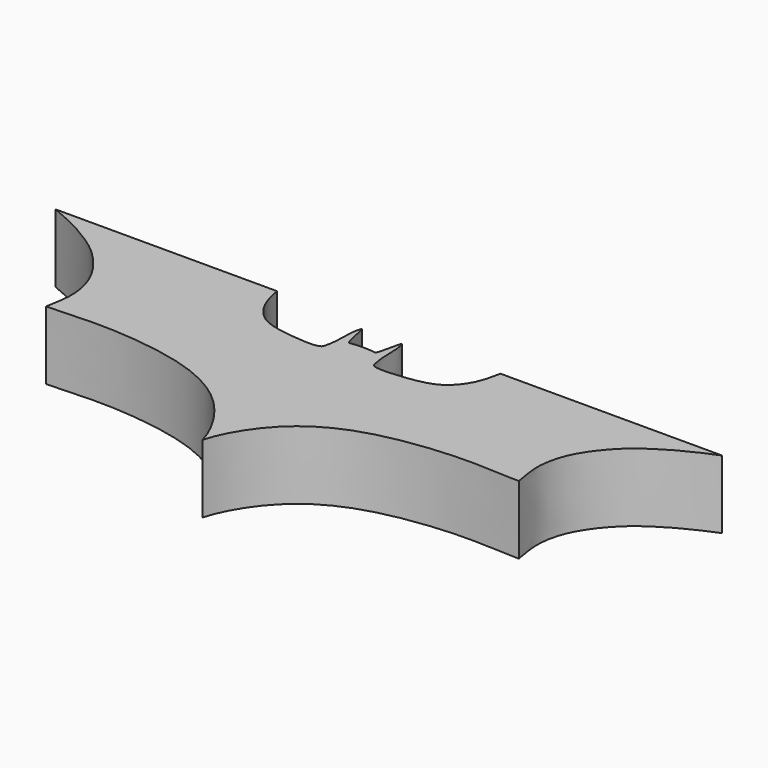
from build123d import *

# Parameters (mm, degrees)
F1_DEPTH = 10


with BuildPart() as f1:
    # F0 (on Top) → F1 (new body)
    with BuildSketch(Plane.XY):
        with BuildLine():
            add(Edge.make_bspline(
                [(-34.5659777522, -2.3010377772), (-34.441690892, -1.2090269011), (-33.7426143908, 1.3021229087), (-34.6099625003, 6.2887083902), (-37.732299485, 10.4337765544), (-40.4965689238, 12.9182984992), (-45.1676660532, 15.6816198367), (-47.6433440327, 16.6521064837), (-48.734344542, 17.1325933188)],
                knots=[0, 0, 0, 0, 0.1504717907, 0.3274056637, 0.505806187, 0.6605615473, 0.844008032, 1, 1, 1, 1], degree=3))
            add(Edge.make_bspline(
                [(-34.5659777522, -2.3010377772), (-29.7742336988, -2.0793164149), (-24.8478324902, -1.8245382393), (-12.9343956026, -3.3284422394), (-4.2994288291, -8.106275212), (-0.6981744502, -14.3344540986), (0, -16.8964266777)],
                knots=[0, 0, 0, 0, 0.2532524451, 0.514284306, 0.7614910609, 1, 1, 1, 1], degree=3))
            add(Edge.make_bspline(
                [(34.5659777522, -2.3010377772), (29.7742336988, -2.0793164149), (24.8478324902, -1.8245382393), (12.9343956026, -3.3284422394), (4.2994288291, -8.106275212), (0.6981744502, -14.3344540986), (0, -16.8964266777)],
                knots=[0, 0, 0, 0, 0.2532524451, 0.514284306, 0.7614910609, 1, 1, 1, 1], degree=3))
            add(Edge.make_bspline(
                [(34.5659777522, -2.3010377772), (34.441690892, -1.2090269011), (33.7426143908, 1.3021229087), (34.6099625003, 6.2887083902), (37.732299485, 10.4337765544), (40.4965689238, 12.9182984992), (45.1676660532, 15.6816198367), (47.6433440327, 16.6521064837), (48.734344542, 17.1325933188)],
                knots=[0, 0, 0, 0, 0.1504717907, 0.3274056637, 0.505806187, 0.6605615473, 0.844008032, 1, 1, 1, 1], degree=3))
            Line((48.734344542, 17.1325933188), (16.3374114782, 17.1325933188))
            add(Edge.make_bspline(
                [(16.3374114782, 17.1325933188), (16.2707590578, 16.8013167715), (16.1028193617, 16.0159047713), (15.5293351039, 13.5894216644), (13.5075885145, 10.9357028955), (11.0943832685, 9.979418199), (8.3278162532, 9.4999515323), (4.2337515187, 9.1916813282), (3.7513867907, 9.7417653506), (3.721309654, 9.7951889602)],
                knots=[0, 0, 0, 0, 0.1002529863, 0.2510752424, 0.4252888894, 0.575274046, 0.7448218724, 0.9396020225, 0.9846016995, 0.9846016995, 0.9846016995, 0.9846016995], degree=3))
            Line((3.721309654, 9.7951889602), (3.6973344953, 9.8154297664))
            add(Edge.make_bspline(
                [(2.932772506, 15.9026999027), (3.018619719, 15.6514358008), (3.2073644933, 15.0990033508), (3.3168408961, 13.9617858734), (3.3565401619, 12.068204215), (3.4100837285, 11.0186767215), (3.599767527, 10.2241220004), (3.6973344953, 9.8154297664)],
                knots=[0, 0, 0, 0, 0.16399089, 0.3605524565, 0.6106599974, 0.7997365931, 1, 1, 1, 1], degree=3))
            add(Edge.make_bspline(
                [(2.932772506, 15.9026999027), (2.8831992541, 15.7815790305), (2.7595296769, 15.4794207803), (2.6079557623, 14.5179694226), (2.311756701, 13.4620564486), (2.1469901884, 12.6659080553), (2.0074066607, 12.3726247092), (1.9479012117, 12.2475959361)],
                knots=[0, 0, 0, 0, 0.1539432383, 0.3840396681, 0.6350969803, 0.8444392514, 1, 1, 1, 1], degree=3))
            add(Edge.make_bspline(
                [(1.9479012117, 12.2475959361), (1.7516233528, 12.2796352379), (1.3532942381, 12.3446562585), (0.7217223004, 12.418893829), (0.2458943028, 12.4186232246), (0, 12.418483384)],
                knots=[0, 0, 0, 0, 0.3194597762, 0.6483162725, 1, 1, 1, 1], degree=3))
            add(Edge.make_bspline(
                [(-1.9479012117, 12.2475959361), (-1.7516233528, 12.2796352379), (-1.3532942381, 12.3446562585), (-0.7217223004, 12.418893829), (-0.2458943028, 12.4186232246), (0, 12.418483384)],
                knots=[0, 0, 0, 0, 0.3194597762, 0.6483162725, 1, 1, 1, 1], degree=3))
            add(Edge.make_bspline(
                [(-2.932772506, 15.9026999027), (-2.8831992541, 15.7815790305), (-2.7595296769, 15.4794207803), (-2.6079557623, 14.5179694226), (-2.311756701, 13.4620564486), (-2.1469901884, 12.6659080553), (-2.0074066607, 12.3726247092), (-1.9479012117, 12.2475959361)],
                knots=[0, 0, 0, 0, 0.1539432383, 0.3840396681, 0.6350969803, 0.8444392514, 1, 1, 1, 1], degree=3))
            add(Edge.make_bspline(
                [(-2.932772506, 15.9026999027), (-3.018619719, 15.6514358008), (-3.2073644933, 15.0990033508), (-3.3168408961, 13.9617858734), (-3.3565401619, 12.068204215), (-3.4100837285, 11.0186767215), (-3.599767527, 10.2241220004), (-3.6973344953, 9.8154297664)],
                knots=[0, 0, 0, 0, 0.16399089, 0.3605524565, 0.6106599974, 0.7997365931, 1, 1, 1, 1], degree=3))
            Line((-3.6973344953, 9.8154297664), (-3.721309654, 9.7951889602))
            add(Edge.make_bspline(
                [(-16.3374114782, 17.1325933188), (-16.2707590578, 16.8013167715), (-16.1028193617, 16.0159047713), (-15.5293351039, 13.5894216644), (-13.5075885145, 10.9357028955), (-11.0943832685, 9.979418199), (-8.3278162532, 9.4999515323), (-4.2337515187, 9.1916813282), (-3.7513867907, 9.7417653506), (-3.721309654, 9.7951889602)],
                knots=[0, 0, 0, 0, 0.1002529863, 0.2510752424, 0.4252888894, 0.575274046, 0.7448218724, 0.9396020225, 0.9846016995, 0.9846016995, 0.9846016995, 0.9846016995], degree=3))
            Line((-16.3374114782, 17.1325933188), (-48.734344542, 17.1325933188))
        make_face()
    extrude(amount=F1_DEPTH)


solid = f1.part
